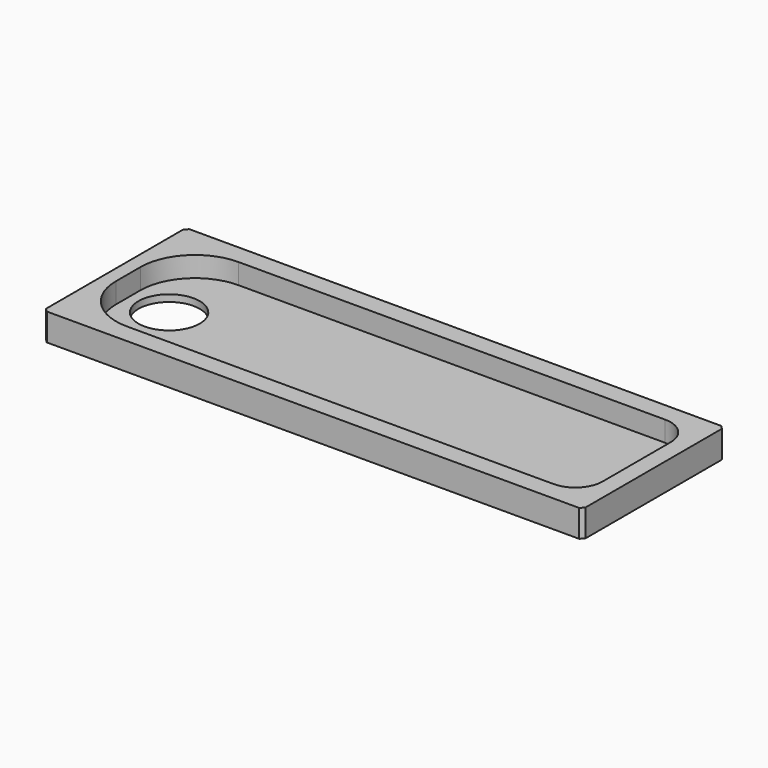
from build123d import *

# Parameters (mm, degrees)
F1_DEPTH = 3
F0_R     = 4.5
F2_DEPTH = 1
F3_SIZE  = 0.5


with BuildPart() as f1:
    # F0 (on Top) → F1 (new body)
    with BuildSketch(Plane.XY):
        Polygon((71.2, 13.05), (-8, 13.1), (-8, -13.1), (71.2, -13.05), align=None)
        with BuildLine():
            ThreePointArc((-6, 2.25), (-3.6568542495, 7.9068542495), (2, 10.25))
            Line((2, 10.25), (64.7, 10.25))
            ThreePointArc((64.7, 10.25), (67.5284271247, 9.0784271247), (68.7, 6.25))
            Line((68.7, 6.25), (68.7, -6.25))
            ThreePointArc((68.7, -6.25), (67.5284271247, -9.0784271247), (64.7, -10.25))
            Line((64.7, -10.25), (2, -10.25))
            ThreePointArc((2, -10.25), (-3.6568542495, -7.9068542495), (-6, -2.25))
            Line((-6, -2.25), (-6, 2.25))
        make_face(mode=Mode.SUBTRACT)
    extrude(amount=F1_DEPTH)

    # F0 (on Top) → F2 (join)
    with BuildSketch(Plane.XY):
        Polygon((71.2, 13.05), (-8, 13.1), (-8, -13.1), (71.2, -13.05), align=None)
        with BuildLine():
            ThreePointArc((-6, 2.25), (-3.6568542495, 7.9068542495), (2, 10.25))
            Line((2, 10.25), (64.7, 10.25))
            ThreePointArc((64.7, 10.25), (67.5284271247, 9.0784271247), (68.7, 6.25))
            Line((68.7, 6.25), (68.7, -6.25))
            ThreePointArc((68.7, -6.25), (67.5284271247, -9.0784271247), (64.7, -10.25))
            Line((64.7, -10.25), (2, -10.25))
            ThreePointArc((2, -10.25), (-3.6568542495, -7.9068542495), (-6, -2.25))
            Line((-6, -2.25), (-6, 2.25))
        make_face(mode=Mode.SUBTRACT)
        with BuildLine():
            Line((64.7, 10.25), (2, 10.25))
            ThreePointArc((2, 10.25), (-3.6568542495, 7.9068542495), (-6, 2.25))
            Line((-6, 2.25), (-6, -2.25))
            ThreePointArc((-6, -2.25), (-3.6568542495, -7.9068542495), (2, -10.25))
            Line((2, -10.25), (64.7, -10.25))
            ThreePointArc((64.7, -10.25), (67.5284271247, -9.0784271247), (68.7, -6.25))
            Line((68.7, -6.25), (68.7, 6.25))
            ThreePointArc((68.7, 6.25), (67.5284271247, 9.0784271247), (64.7, 10.25))
        make_face()
        Circle(F0_R, mode=Mode.SUBTRACT)
    extrude(amount=-F2_DEPTH)

    # F3
    f3_edges = [f1.edges().sort_by_distance(p)[0] for p in [
        (-8, -13.1, 1),
        (-8, 13.1, 1),
        (71.2, -13.05, 1),
        (71.2, 13.05, 1),
    ]]
    chamfer(f3_edges, length=F3_SIZE)


solid = f1.part
